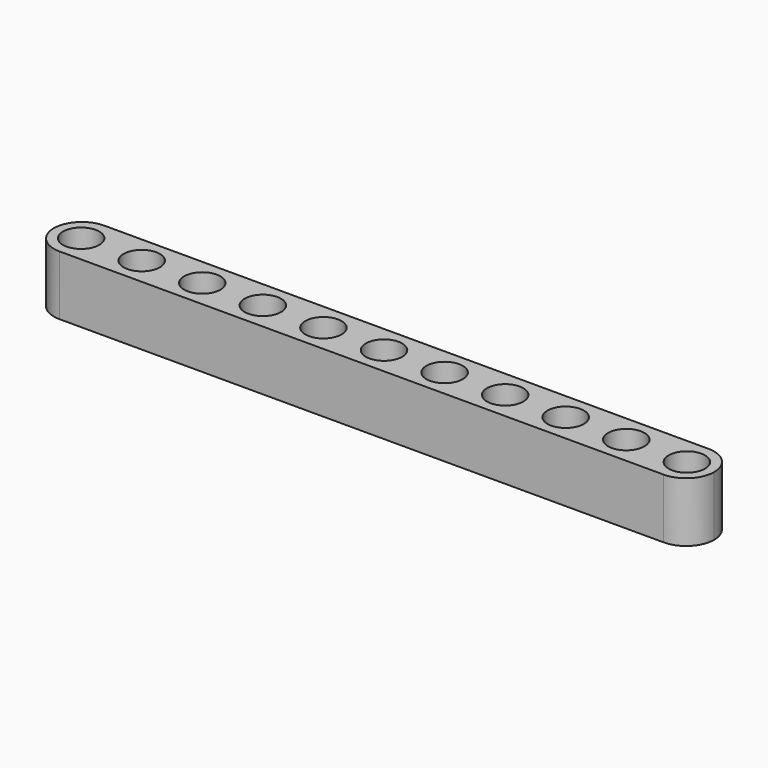
from build123d import *

# Parameters (mm, degrees)
F0_R        = 2.4
F1_DEPTH    = 7.88
F2_T1_DEPTH = 26.405


# Not quite as in the source:
# - a fillet or chamfer that OpenCascade refuses, or shapes differently, is made with other operations: its cross-section is extruded or revolved along the edge and cut away or added


with BuildPart() as f1:
    # F0 (on Top) → F1 (new body)
    with BuildSketch(Plane.XY):
        Polygon((14.8854916829, 1.6058013724), (-28.7195083171, 1.6058013724), (-72.3245083171, 1.6058013724), (-72.3245083171, -2.0891986276), (-72.3245083171, -5.7841986276), (-28.7195083171, -5.7841986276), (14.8854916829, -5.7841986276), (14.8854916829, -2.0891986276), align=None)
        with Locations((-68.7195083171, -2.0891986276)):
            Circle(F0_R, mode=Mode.SUBTRACT)
        with Locations((-60.7195083171, -2.0891986276)):
            Circle(F0_R, mode=Mode.SUBTRACT)
        with Locations((-52.7195083171, -2.0891986276)):
            Circle(F0_R, mode=Mode.SUBTRACT)
        with Locations((-44.7195083171, -2.0891986276)):
            Circle(F0_R, mode=Mode.SUBTRACT)
        with Locations((-36.7195083171, -2.0891986276)):
            Circle(F0_R, mode=Mode.SUBTRACT)
        with BuildLine():
            ThreePointArc((-28.7195083171, -4.4891986276), (-31.1195083171, -2.0891986276), (-28.7195083171, 0.3108013724))
            ThreePointArc((-28.7195083171, 0.3108013724), (-26.3195083171, -2.0891986276), (-28.7195083171, -4.4891986276))
        make_face(mode=Mode.SUBTRACT)
        with Locations((-20.7195083171, -2.0891986276)):
            Circle(F0_R, mode=Mode.SUBTRACT)
        with Locations((-12.7195083171, -2.0891986276)):
            Circle(F0_R, mode=Mode.SUBTRACT)
        with Locations((-4.7195083171, -2.0891986276)):
            Circle(F0_R, mode=Mode.SUBTRACT)
        with Locations((3.2804916829, -2.0891986276)):
            Circle(F0_R, mode=Mode.SUBTRACT)
        with Locations((11.2804916829, -2.0891986276)):
            Circle(F0_R, mode=Mode.SUBTRACT)
    extrude(amount=F1_DEPTH)

    # F2: fillet of radius 3.705 on 4 edges, made by hand

    # F2_s2 → F2_t1 (cut)
    with BuildSketch(Plane.XY.offset(-9.2625)):
        with BuildLine():
            ThreePointArc((11.1804916829, 1.6058013724), (13.8003223072, 0.5206319967), (14.8854916829, -2.0991986276))
            Line((14.8854916829, -2.0991986276), (14.8854916829, 1.6058013724))
            Line((14.8854916829, 1.6058013724), (11.1804916829, 1.6058013724))
        make_face()
        with BuildLine():
            ThreePointArc((11.1804916829, -5.7841986276), (13.8003223072, -4.6990292519), (14.8854916829, -2.0791986276))
            Line((14.8854916829, -2.0791986276), (14.8854916829, -5.7841986276))
            Line((14.8854916829, -5.7841986276), (11.1804916829, -5.7841986276))
        make_face()
        with BuildLine():
            ThreePointArc((-68.6195083171, 1.6058013724), (-71.2393389413, 0.5206319967), (-72.3245083171, -2.0991986276))
            Line((-72.3245083171, -2.0991986276), (-72.3245083171, 1.6058013724))
            Line((-72.3245083171, 1.6058013724), (-68.6195083171, 1.6058013724))
        make_face()
        with BuildLine():
            ThreePointArc((-68.6195083171, -5.7841986276), (-71.2393389413, -4.6990292519), (-72.3245083171, -2.0791986276))
            Line((-72.3245083171, -2.0791986276), (-72.3245083171, -5.7841986276))
            Line((-72.3245083171, -5.7841986276), (-68.6195083171, -5.7841986276))
        make_face()
    extrude(amount=F2_T1_DEPTH, mode=Mode.SUBTRACT)


solid = f1.part
